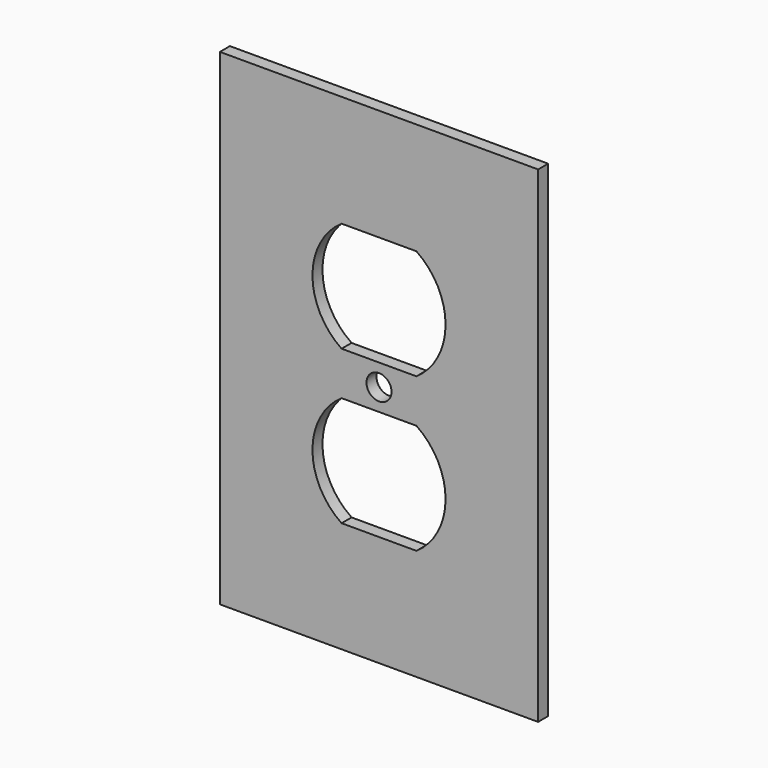
from build123d import *

# Parameters (mm, degrees)
F0_W     = 80.772
F0_H     = 123.444
F0_R     = 3.175
F1_DEPTH = 3.175


# Not quite as in the source:
# - ends of sketch curves that miss each other by under 0.0002 mm in the source are joined


with BuildPart() as f1:
    # F0 (on Front) → F1 (new body)
    with BuildSketch(Plane.XZ):
        Rectangle(F0_W, F0_H)
        with BuildLine():
            ThreePointArc((-9.4932913315, -33.5419135021), (-16.889821539, -19.5719126303), (-9.4932913315, -5.6019117584))
            Line((-9.4932913315, -5.6019117584), (9.495647661, -5.6019126303))
            ThreePointArc((9.495647661, -5.6019126303), (16.892178461, -19.5719126303), (9.4956482536, -33.5419135021))
            Line((9.4956482536, -33.5419135021), (-9.4932913315, -33.5419135021))
        make_face(mode=Mode.SUBTRACT)
        with Locations((0.001178461, -0.0774126303)):
            Circle(F0_R, mode=Mode.SUBTRACT)
        with BuildLine():
            ThreePointArc((-9.4932913315, 5.4470864979), (-16.889821539, 19.4170873697), (-9.4932913315, 33.3870882416))
            Line((-9.4932913315, 33.3870882416), (9.495647661, 33.3870873697))
            ThreePointArc((9.495647661, 33.3870873697), (16.892178461, 19.4170873697), (9.4956482536, 5.4470864979))
            Line((9.4956482536, 5.4470864979), (-9.4932913315, 5.4470864979))
        make_face(mode=Mode.SUBTRACT)
    extrude(amount=F1_DEPTH)


solid = f1.part
